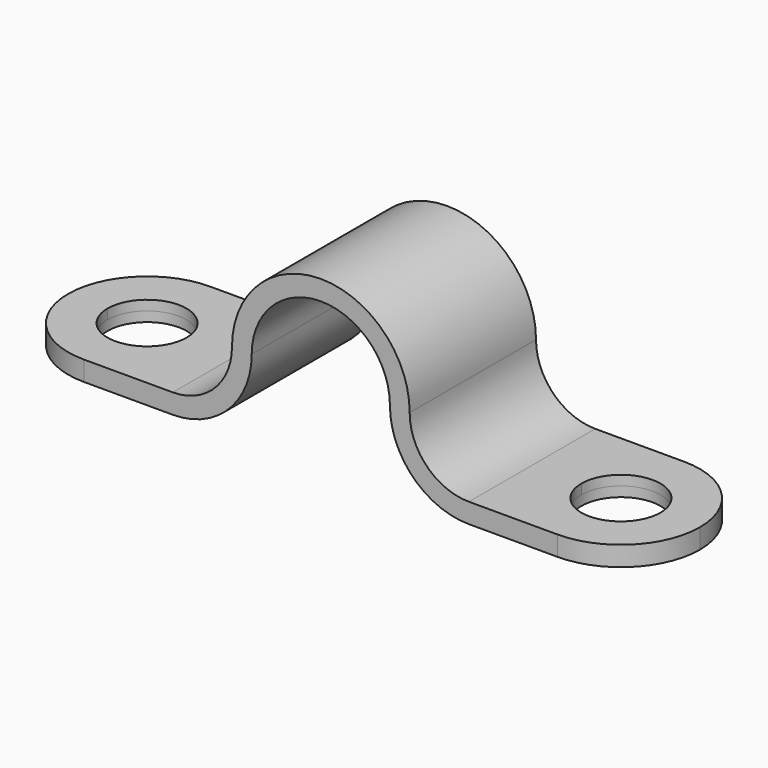
from build123d import *

# Parameters (mm, degrees)
F1_DEPTH = 6.35
F2_R     = 6.34999
F4_D     = 6.35
F4_DEPTH = 12.701
F5_D     = 6.35


# Not quite as in the source:
# - a fillet or chamfer is up to 0.001 mm smaller than in the source, because OpenCascade refuses the exact size


with BuildPart() as f1:
    # F0 (on Front) → F1 (new body, symmetric)
    with BuildSketch(Plane.XZ):
        with BuildLine():
            Line((-11.90625, 0.79375), (-25.4, 0.79375))
            Line((-25.4, 0.79375), (-25.4, -0.79375))
            Line((-25.4, -0.79375), (-11.90625, -0.79375))
            ThreePointArc((-11.90625, -0.79375), (-7.4161219395, 1.0661219395), (-5.55625, 5.55625))
            ThreePointArc((-5.55625, 5.55625), (0, 11.1125), (5.55625, 5.55625))
            ThreePointArc((5.55625, 5.55625), (7.4161219395, 1.0661219395), (11.90625, -0.79375))
            Line((11.90625, -0.79375), (25.4, -0.79375))
            Line((25.4, -0.79375), (25.4, 0.79375))
            Line((25.4, 0.79375), (11.90625, 0.79375))
            ThreePointArc((11.90625, 0.79375), (8.5386539546, 2.1886539546), (7.14375, 5.55625))
            ThreePointArc((7.14375, 5.55625), (0, 12.7), (-7.14375, 5.55625))
            ThreePointArc((-7.14375, 5.55625), (-8.5386539546, 2.1886539546), (-11.90625, 0.79375))
        make_face()
    extrude(amount=F1_DEPTH, both=True)

    # F2 (radius 6.35 in the source; OpenCascade refuses exactly that, so slightly less here)
    f2_edges = [f1.edges().sort_by_distance(p)[0] for p in [
        (25.4, -6.35, 0),
        (25.4, 6.35, 0),
        (-25.4, -6.35, 0),
        (-25.4, 6.35, 0),
    ]]
    fillet(f2_edges, radius=F2_R)

    # F4 (through all, one way)
    with BuildSketch(Plane(origin=(0, 0, 0), x_dir=(1, 0, 0), z_dir=(0, 0, -1))):
        with Locations((-19.05, 0), (19.05, 0)):
            Circle(F4_D / 2)
    extrude(amount=-F4_DEPTH, mode=Mode.SUBTRACT)

    # F5 (through all)
    with Locations(Plane.XY):
        with Locations((-19.05, 0), (19.05, 0)):
            Hole(F5_D / 2)


solid = f1.part
